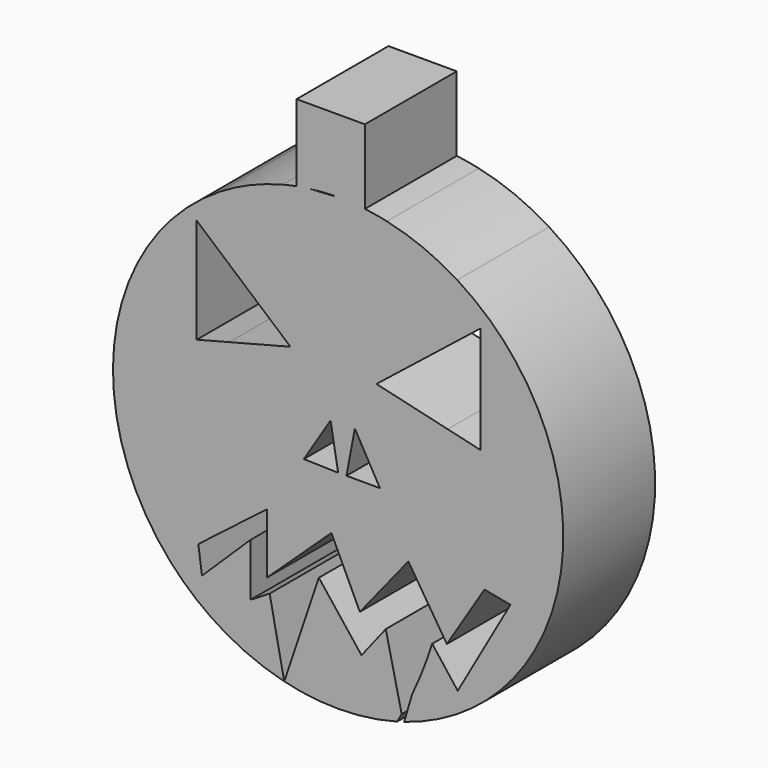
from build123d import *

# Parameters (mm, degrees)
F1_DEPTH = 25.4


with BuildPart() as f1:
    # F0 (on Front) → F1 (new body)
    with BuildSketch(Plane.XZ):
        with BuildLine():
            ThreePointArc((32.6782151723, -37.5764677752), (45.3165071723, -20.6463278819), (49.7981593767, 0))
            ThreePointArc((49.7981593767, 0), (43.5428138182, 24.1636098732), (26.3482949877, 42.2566447857))
            ThreePointArc((26.3482949877, 42.2566447857), (42.3711325354, 3.3595819889), (32.6782151723, -37.5764677752))
        make_face()
        with BuildLine():
            ThreePointArc((32.6782151723, -37.5764677752), (42.3711325354, 3.3595819889), (26.3482949877, 42.2566447857))
            ThreePointArc((26.3482949877, 42.2566447857), (18.8375502119, 46.0977589403), (10.7862166768, 48.6159871555))
            ThreePointArc((10.7862166768, 48.6159871555), (16.6744949948, 37.7627754895), (21.092116807, 26.232439738))
            Line((21.092116807, 26.232439738), (31.447738409, 34.4624482095))
            Line((31.447738409, 34.4624482095), (31.447738409, 10.8348272407))
            Line((31.447738409, 10.8348272407), (24.2378107652, 12.519994233))
            ThreePointArc((24.2378107652, 12.519994233), (25.1538459711, -6.9642629039), (22.0360332318, -26.2192529167))
            Line((22.0360332318, -26.2192529167), (24.0468364209, -29.366614297))
            Line((24.0468364209, -29.366614297), (32.37285465, -16.0449128598))
            Line((32.37285465, -16.0449128598), (38.1085574627, -17.1593967825))
            Line((38.1085574627, -17.1593967825), (26.4521297067, -37.6942455769))
            Line((26.4521297067, -37.6942455769), (20.8098572617, -30.369653677))
            ThreePointArc((20.8098572617, -30.369653677), (18.7701982142, -36.0902111883), (16.3660323787, -41.6673945191))
            Line((16.3660323787, -41.6673945191), (14.5917575654, -47.6123648694))
            ThreePointArc((14.5917575654, -47.6123648694), (24.1617960482, -43.5438203311), (32.6782151723, -37.5764677752))
        make_face()
        with BuildLine():
            ThreePointArc((21.092116807, 26.232439738), (16.6744949948, 37.7627754895), (10.7862166768, 48.6159871555))
            ThreePointArc((10.7862166768, 48.6159871555), (8.3607166752, 49.0912934642), (5.9146205895, 49.4456665502))
            ThreePointArc((5.9146205895, 49.4456665502), (2.9625575062, 49.70995806), (0, 49.7981593767))
            Line((0, 49.7981593767), (0, -3.8344066124))
            Line((0, -3.8344066124), (0, -19.1923552025))
            Line((0, -19.1923552025), (4.8044845462, -29.366614297))
            Line((4.8044845462, -29.366614297), (15.5357960612, -16.0449128598))
            Line((15.5357960612, -16.0449128598), (22.0360332318, -26.2192529167))
            ThreePointArc((22.0360332318, -26.2192529167), (25.1538459711, -6.9642629039), (24.2378107652, 12.519994233))
            Line((24.2378107652, 12.519994233), (8.4741063403, 16.204424325))
            Line((8.4741063403, 16.204424325), (21.092116807, 26.232439738))
        make_face()
        Polygon((9.245027788, -3.8344066124), (1.8441228895, -3.8344066124), (3.6943492014, 5.9712096117), align=None, mode=Mode.SUBTRACT)
        with BuildLine():
            ThreePointArc((0, 49.7981593767), (2.9625575062, 49.70995806), (5.9146205895, 49.4456665502))
            Line((5.9146205895, 49.4456665502), (5.9146205895, 65.9195636089))
            Line((5.9146205895, 65.9195636089), (3.1392811798, 65.9195636089))
            Line((3.1392811798, 65.9195636089), (0, 65.9195636089))
            Line((0, 65.9195636089), (0, 49.7981593767))
        make_face()
        with BuildLine():
            Line((0, -3.8344066124), (0, 49.7981593767))
            Line((0, 49.7981593767), (-6.296872627, 49.398442004))
            ThreePointArc((-6.296872627, 49.398442004), (-7.744154843, 49.1923240259), (-9.1847632403, 48.9438126991))
            ThreePointArc((-9.1847632403, 48.9438126991), (-10.7192794325, 48.6307898944), (-12.2431936307, 48.2696683957))
            ThreePointArc((-12.2431936307, 48.2696683957), (-17.0201913462, 37.3889257354), (-20.9051760668, 26.1587359893))
            Line((-20.9051760668, 26.1587359893), (-10.5523923412, 17.2587409616))
            Line((-10.5523923412, 17.2587409616), (-24.0617127081, 13.7618819272))
            ThreePointArc((-24.0617127081, 13.7618819272), (-26.7647104228, -5.37655391), (-26.9402397571, -24.7041277979))
            Line((-26.9402397571, -24.7041277979), (-15.7330241054, -16.0449128598))
            Line((-15.7330241054, -16.0449128598), (-15.7330241054, -29.366614297))
            Line((-15.7330241054, -29.366614297), (-1.4862839598, -16.0449128598))
            Line((-1.4862839598, -16.0449128598), (0, -19.1923552025))
            Line((0, -19.1923552025), (0, -3.8344066124))
        make_face()
        Polygon((-1.6713063233, 5.7866196148), (0, -3.8344066124), (-7.5920294039, -3.6490550265), align=None, mode=Mode.SUBTRACT)
        with BuildLine():
            ThreePointArc((-6.296872627, 49.398442004), (-3.1547733222, 49.6981295683), (0, 49.7981593767))
            Line((0, 49.7981593767), (0, 65.9195636089))
            Line((0, 65.9195636089), (-3.1484363135, 65.9195636089))
            Line((-3.1484363135, 65.9195636089), (-6.296872627, 65.9195636089))
            Line((-6.296872627, 65.9195636089), (-6.296872627, 49.398442004))
        make_face()
        with BuildLine():
            ThreePointArc((-9.1847632403, 48.9438126991), (-7.744154843, 49.1923240259), (-6.296872627, 49.398442004))
            Line((-6.296872627, 49.398442004), (-6.296872627, 65.9195636089))
            Line((-6.296872627, 65.9195636089), (-9.1847632403, 65.9195636089))
            Line((-9.1847632403, 65.9195636089), (-9.1847632403, 48.9438126991))
        make_face()
        with BuildLine():
            ThreePointArc((-24.7076516572, -43.2364270829), (-18.4904087752, -46.2380953396), (-11.9177707221, -48.3510436115))
            Line((-11.9177707221, -48.3510436115), (-15.1432544542, -32.3012661093))
            Line((-15.1432544542, -32.3012661093), (-19.4334760308, -34.9169038236))
            Line((-19.4334760308, -34.9169038236), (-19.4334760308, -23.2604946941))
            Line((-19.4334760308, -23.2604946941), (-26.5274317789, -30.1849724934))
            ThreePointArc((-26.5274317789, -30.1849724934), (-25.7634681206, -36.7310464832), (-24.7076516572, -43.2364270829))
        make_face()
        with BuildLine():
            ThreePointArc((-20.9051760668, 26.1587359893), (-17.0201913462, 37.3889257354), (-12.2431936307, 48.2696683957))
            ThreePointArc((-12.2431936307, 48.2696683957), (-19.4406831361, 45.8466630902), (-26.1860345343, 42.3573874628))
            ThreePointArc((-26.1860345343, 42.3573874628), (-41.8830905525, 6.0124933669), (-37.0441602385, -33.2804277246))
            ThreePointArc((-37.0441602385, -33.2804277246), (-31.2746230818, -38.7524789968), (-24.7076516572, -43.2364270829))
            ThreePointArc((-24.7076516572, -43.2364270829), (-25.7634681206, -36.7310464832), (-26.5274317789, -30.1849724934))
            Line((-26.5274317789, -30.1849724934), (-30.1115038325, -33.6834193751))
            Line((-30.1115038325, -33.6834193751), (-30.925318067, -27.7831842472))
            Line((-30.925318067, -27.7831842472), (-26.9402397571, -24.7041277979))
            ThreePointArc((-26.9402397571, -24.7041277979), (-26.7647104228, -5.37655391), (-24.0617127081, 13.7618819272))
            Line((-24.0617127081, 13.7618819272), (-31.2749259174, 11.8947569281))
            Line((-31.2749259174, 11.8947569281), (-31.2749259174, 35.0733163144))
            Line((-31.2749259174, 35.0733163144), (-20.9051760668, 26.1587359893))
        make_face()
        with BuildLine():
            ThreePointArc((-37.0441602385, -33.2804277246), (-41.8830905525, 6.0124933669), (-26.1860345343, 42.3573874628))
            ThreePointArc((-26.1860345343, 42.3573874628), (-49.292840802, 7.0761941024), (-37.0441602385, -33.2804277246))
        make_face()
    extrude(amount=F1_DEPTH)


with BuildPart() as f1b:
    # F0 (on Front) → F1, piece 2 (new body)
    with BuildSketch(Plane.XZ):
        with BuildLine():
            ThreePointArc((0, -49.7981593767), (6.5886259942, -49.3603756551), (13.0614086221, -48.0547217463))
            ThreePointArc((13.0614086221, -48.0547217463), (13.5613311897, -47.1614128137), (14.0515134569, -46.2627222288))
            Line((14.0515134569, -46.2627222288), (10.5401859619, -30.8488430455))
            Line((10.5401859619, -30.8488430455), (5.1745297387, -37.6942455769))
            Line((5.1745297387, -37.6942455769), (0, -31.0988395126))
            Line((0, -31.0988395126), (0, -49.7981593767))
        make_face()
        with BuildLine():
            ThreePointArc((-11.9177707221, -48.3510436115), (-6.0026536428, -49.4350566557), (0, -49.7981593767))
            Line((0, -49.7981593767), (0, -31.0988395126))
            Line((0, -31.0988395126), (-4.2616231367, -25.6670154631))
            Line((-4.2616231367, -25.6670154631), (-11.9177707221, -48.3510436115))
        make_face()
    extrude(amount=F1_DEPTH)


solid = Compound([f1.part, f1b.part])
